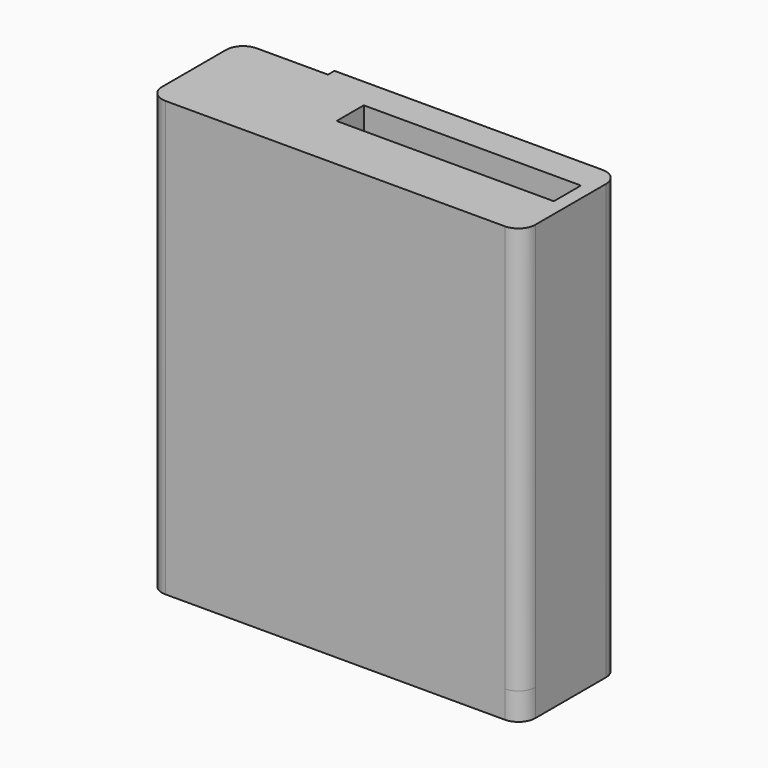
from build123d import *

# Parameters (mm, degrees)
F1_DEPTH  = 60
F3_DEPTH  = 12
F4_R      = 2.5
F5_DEPTH  = 4
F6_W      = 5
F6_H      = 5
F7_DEPTH  = 52
F8_W      = 20
F8_H      = 2
F9_DEPTH  = 17
F12_DEPTH = 4
F14_W     = 19.9
F14_H     = 2
F15_DEPTH = 0.5


# Not quite as in the source:
# - a feature names something its author has since deleted; it is built from what else it names


with BuildPart() as f1:
    # F0 (on Top) → F1 (new body)
    with BuildSketch(Plane.XY):
        Polygon((-8, 0), (0, 0), (0, 8), (-8, 8), (-13, 8), (-13, -6.8), (-13, -8.8), (42, -8.8), (42, 9.2), (10, 9.2), (10, 7.2), (40, 7.2), (40, -6.8), (0, -6.8), (0, -1.8), (-8, -1.8), align=None)
    extrude(amount=F1_DEPTH)

    # F2 (on face) → F3 (join)
    with BuildSketch(Plane.XY.offset(60)):
        Polygon((40, -0.4), (8, -0.4), (8, 4.6), (40, 4.6), (40, 7.2), (10, 7.2), (10, 9.2), (0, 9.2), (0, 8), (0, 0), (-8, 0), (-8, -1.8), (0, -1.8), (0, -6.8), (40, -6.8), align=None)
    extrude(amount=-F3_DEPTH)

    # F4
    f4_edges = [f1.edges().sort_by_distance(p)[0] for p in [
        (42, 9.2, 30),
        (42, -8.8, 30),
        (-13, -8.8, 30),
        (-13, 8, 30),
    ]]
    fillet(f4_edges, radius=F4_R)

    # F5 (add): a face of the model
    f5_faces = [f1.faces().sort_by_distance(p)[0] for p in [
        (-5.25, 7.4212945482, 0),
    ]]
    extrude(f5_faces, amount=F5_DEPTH)

    # F6 (on face) → F7 (join)
    with BuildSketch(Plane(origin=(0, 0, 48), x_dir=(1, 0, 0), z_dir=(0, 0, -1))):
        with Locations((37.5, 4.3)):
            Rectangle(F6_W, F6_H)
    extrude(amount=F7_DEPTH)

    # F8 (on face) → F9 (cut)
    with BuildSketch(Plane(origin=(0, 9.2, 0), x_dir=(-1, 0, 0), z_dir=(0, 1, 0))):
        with Locations((-25, -1)):
            Rectangle(F8_W, F8_H)
    extrude(amount=-F9_DEPTH, mode=Mode.SUBTRACT)


with BuildPart() as f12:
    # F11 (on face) → F12 (new body)
    with BuildSketch(Plane(origin=(0, 0, -4), x_dir=(1, 0, 0), z_dir=(0, 0, -1))):
        Polygon((9.9, -9.1), (9.9, -7.1), (39.9, -7.1), (39.9, 1.7), (34.9, 1.7), (34.9, 6.7), (0.1, 6.7), (0.1, 1.7), (-7.9, 1.7), (-7.9, 0.1), (0.1, 0.1), (0.1, -0.2000001237), (0.1, -9.1), align=None)
    extrude(amount=-F12_DEPTH)

    # F14 (on face) → F15 (join)
    with BuildSketch(Plane.XZ.offset(6.7)):
        with Locations((24.95, -1)):
            Rectangle(F14_W, F14_H)
    extrude(amount=F15_DEPTH)


solid = Compound([f1.part, f12.part])
